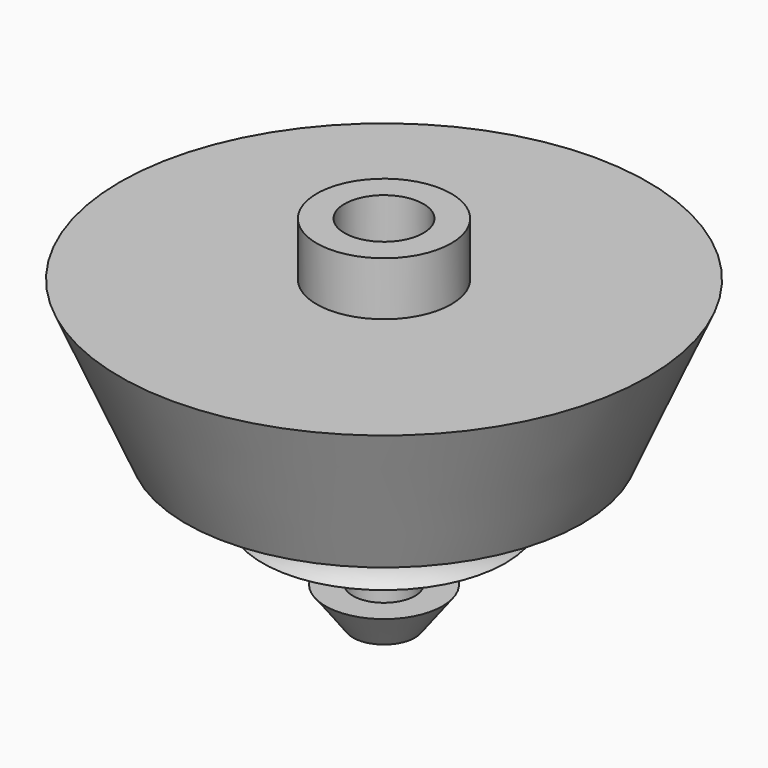
from build123d import *

# Parameters (mm, degrees)
F2_R     = 1.5728770132
F3_DEPTH = 20.955
F4_R     = 4.7463390005
F5_DEPTH = 9.525


# Not quite as in the source:
# - a feature names something its author has since deleted; it is built from what else it names


with BuildPart() as f1:
    # F0 (on Front) → F1 (revolve)
    with BuildSketch(Plane.XZ):
        with BuildLine():
            Line((0, 20.9652427214), (0, 6.7289513536))
            Line((0, 6.7289513536), (0, -22.2147572786))
            Line((0, -22.2147572786), (3.7280632295, -22.2147572786))
            Line((3.7280632295, -22.2147572786), (7.0464526415, -17.7902411669))
            Line((7.0464526415, -17.7902411669), (3.7280632295, -17.7902411669))
            Line((3.7280632295, -17.7902411669), (3.7280632295, -14.6562093869))
            Line((3.7280632295, -14.6562093869), (14.6050014645, -10.7847582549))
            ThreePointArc((14.6050014645, -10.7847582549), (13.3991858149, -6.7201295533), (16.2641917467, -3.5949193407))
            Line((16.2641917467, -3.5949193407), (23.8227405697, -3.5949193407))
            Line((23.8227405697, -3.5949193407), (31.75, 14.5086767152))
            Line((31.75, 14.5086767152), (14.6050014645, 14.5086767152))
            Line((14.6050014645, 14.5086767152), (8.0961844996, 14.5086767152))
            Line((8.0961844996, 14.5086767152), (8.0961844996, 20.9652427214))
            Line((8.0961844996, 20.9652427214), (0, 20.9652427214))
        make_face()
    revolve(axis=Axis((0, 0, -7.7429029625), (0, 0, -1)))

    # F2 (on face) → F3 (cut)
    with BuildSketch(Plane(origin=(0, 0, -22.2147572786), x_dir=(1, 0, 0), z_dir=(0, 0, -1))):
        Circle(F2_R)
    extrude(amount=-F3_DEPTH, mode=Mode.SUBTRACT)

    # F4 (on face) → F5 (cut)
    with BuildSketch(Plane.XY.offset(20.9652427214)):
        Circle(F4_R)
    extrude(amount=-F5_DEPTH, mode=Mode.SUBTRACT)


solid = f1.part
